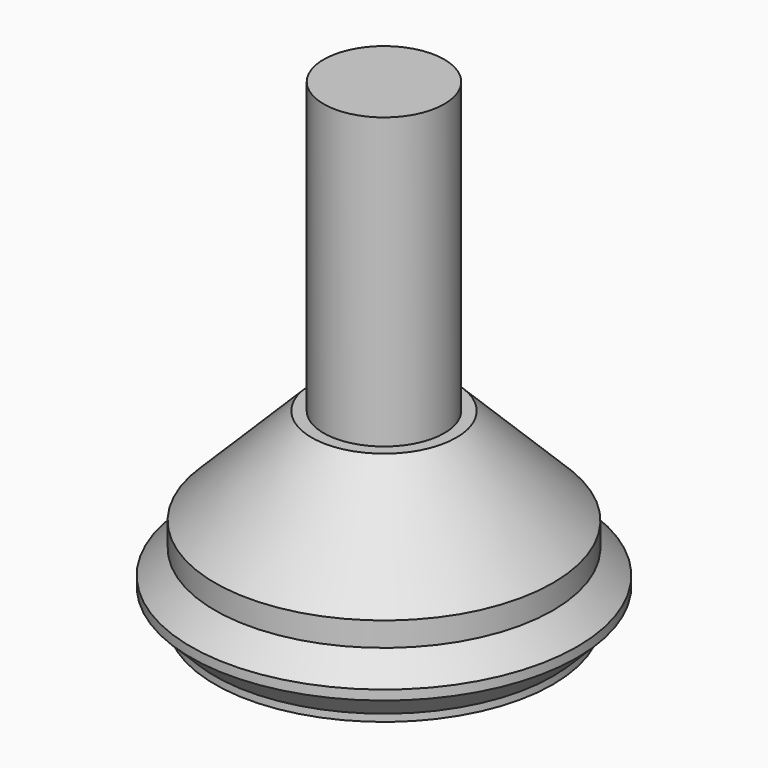
from build123d import *

# Parameters (mm, degrees)
F0_R     = 35
F0_R_2   = 32.5
F1_DEPTH = 40
F2_START = 20
F0_R_3   = 12.5
F2_DEPTH = 20
F3_START = 39
F3_DEPTH = 61
F4_SIZE  = 20
F5_SIZE  = 18.99999
F6_START = 3
F0_R_4   = 40
F6_DEPTH = 12
F7_SIZE  = 4.99999
F8_DEPTH = 1.5


# Not quite as in the source:
# - a fillet or chamfer is up to 0.001 mm smaller than in the source, because OpenCascade refuses the exact size


with BuildPart() as f1:
    # F0 (on Top) → F1 (new body)
    with BuildSketch(Plane.XY):
        Circle(F0_R)
        Circle(F0_R_2, mode=Mode.SUBTRACT)
    extrude(amount=F1_DEPTH)

    # F0 (on Top) → F2 (join)
    with BuildSketch(Plane.XY.offset(F2_START)):
        Circle(F0_R_2)
        Circle(F0_R_3, mode=Mode.SUBTRACT)
    extrude(amount=F2_DEPTH)

    # F0 (on Top) → F3 (join)
    with BuildSketch(Plane.XY.offset(F3_START)):
        Circle(F0_R_3)
    extrude(amount=F3_DEPTH)

    # F4
    f4_edges = [f1.edges().sort_by_distance(p)[0] for p in [
        (-35, 0, 40),
    ]]
    chamfer(f4_edges, length=F4_SIZE)

    # F5 (size 19 in the source; OpenCascade refuses exactly that, so slightly less here)
    f5_edges = [f1.edges().sort_by_distance(p)[0] for p in [
        (-12.5, 0, 20),
    ]]
    chamfer(f5_edges, length=F5_SIZE)

    # F0 (on Top) → F6 (join)
    with BuildSketch(Plane.XY.offset(F6_START)):
        Circle(F0_R_4)
        Circle(F0_R, mode=Mode.SUBTRACT)
    extrude(amount=F6_DEPTH)

    # F7 (size 5 in the source; OpenCascade refuses exactly that, so slightly less here)
    f7_edges = [f1.edges().sort_by_distance(p)[0] for p in [
        (-40, 0, 3),
        (-40, 0, 15),
    ]]
    chamfer(f7_edges, length=F7_SIZE)

    # F8 (cut): a face of the model
    f8_faces = [f1.faces().sort_by_distance(p)[0] for p in [
        (-34.0100505063, 0, 0),
    ]]
    extrude(f8_faces, amount=-F8_DEPTH, mode=Mode.SUBTRACT)


solid = f1.part
